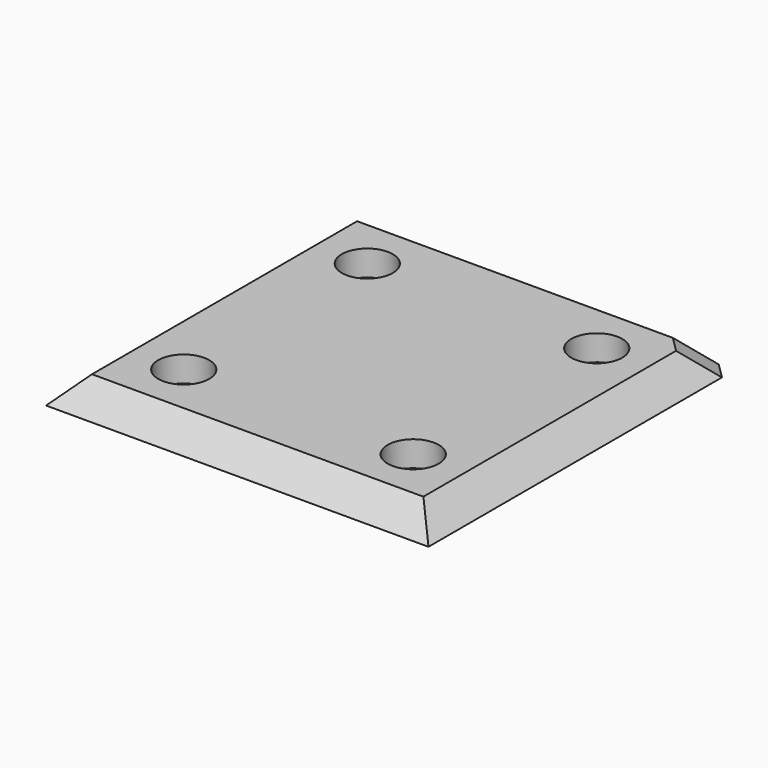
from build123d import *

# Parameters (mm, degrees)
F0_W        = 76.2
F0_H        = 76.2
F1_DEPTH    = 5.08
F2_R        = 5.08
F3_DEPTH    = 25.4
F4_SIZE     = 5.07999
F5_T1_DEPTH = 21.9411964155


# Not quite as in the source:
# - a fillet or chamfer that OpenCascade refuses, or shapes differently, is made with other operations: its cross-section is extruded or revolved along the edge and cut away or added
# - a fillet or chamfer is up to 0.001 mm smaller than in the source, because OpenCascade refuses the exact size


with BuildPart() as f1:
    # F0 (on Top) → F1 (new body)
    with BuildSketch(Plane.XY):
        with Locations((38.1, 38.1)):
            Rectangle(F0_W, F0_H)
    extrude(amount=F1_DEPTH)

    # F2 (on face) → F3 (cut)
    with BuildSketch(Plane.XY.offset(5.08)):
        with Locations((15.24, 60.96)):
            Circle(F2_R)
        with Locations((60.96, 60.96)):
            Circle(F2_R)
        with Locations((15.24, 15.24)):
            Circle(F2_R)
        with Locations((60.96, 15.24)):
            Circle(F2_R)
    extrude(amount=-F3_DEPTH, mode=Mode.SUBTRACT)

    # F4 (size 5.08 in the source; OpenCascade refuses exactly that, so slightly less here)
    f4_edges = [f1.edges().sort_by_distance(p)[0] for p in [
        (38.1, 76.2, 5.08),
        (0, 38.1, 5.08),
        (76.2, 38.1, 5.08),
        (38.1, 0, 5.08),
    ]]
    chamfer(f4_edges, length=F4_SIZE)

    # F5: chamfer of 2.54 on 1 edges, made by hand

    # F5_s2 → F5_t1 (cut)
    with BuildSketch(Plane(origin=(54.5938794951, 54.5938794951, -54.5938794951), x_dir=(0.7071067812, -0.7071067812, 0), z_dir=(-0.5773502692, -0.5773502692, 0.5773502692))):
        Polygon((-2.1997045256, 60.9470476317), (2.1997045256, 60.9470476317), (0, 62.2170476317), align=None)
    extrude(amount=F5_T1_DEPTH, mode=Mode.SUBTRACT)


solid = f1.part
